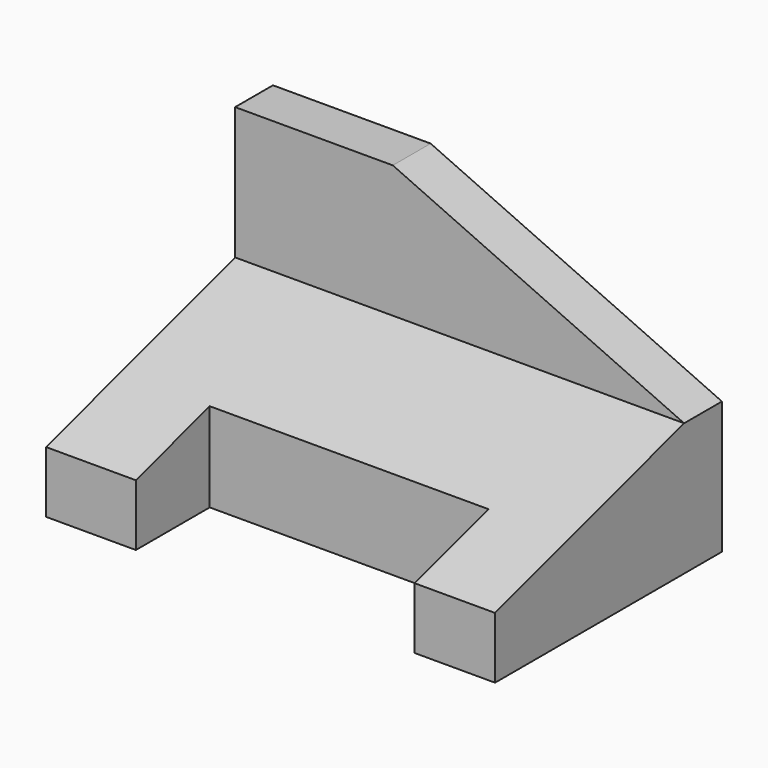
from build123d import *

# Parameters (mm, degrees)
F1_DEPTH = 95
F4_DEPTH = 25
F3_W     = 59
F3_H     = 19.5249739359
F5_DEPTH = 25


# Not quite as in the source:
# - a feature names something its author has since deleted; it is built from what else it names


with BuildPart() as f1:
    # F0 (on Right) → F1 (new body)
    with BuildSketch(Plane.YZ):
        Polygon((-37.6999974251, 2.400000114), (22.3000025749, 2.400000114), (22.3000025749, 58.400000114), (12.3000025749, 58.400000114), (12.3000025749, 30.400000114), (-37.6999974251, 15.400000114), align=None)
    extrude(amount=F1_DEPTH)

    # F2 (on face) → F4 (cut)
    with BuildSketch(Plane.XZ.offset(-12.3000025749)):
        Polygon((95, 58.400000114), (33.3666242659, 58.400000114), (95, 30.400000114), align=None)
    extrude(amount=-F4_DEPTH, mode=Mode.SUBTRACT)

    # F3 (on face) → F5 (cut)
    with BuildSketch(Plane(origin=(0, 0, 2.400000114), x_dir=(1, 0, 0), z_dir=(0, 0, -1))):
        with Locations((48.5, 27.9375104571)):
            Rectangle(F3_W, F3_H)
    extrude(amount=-F5_DEPTH, mode=Mode.SUBTRACT)


solid = f1.part
